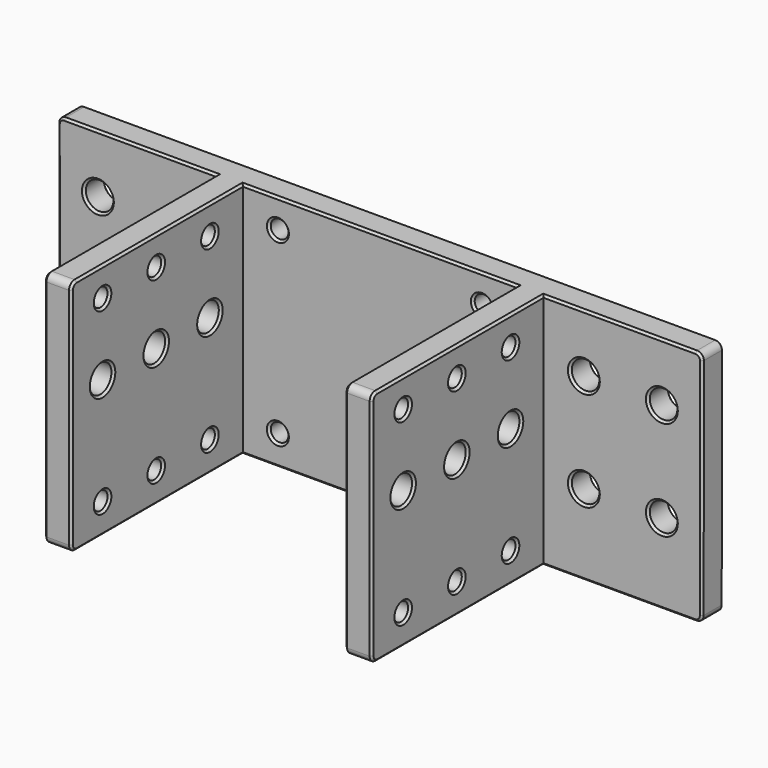
from build123d import *

# Parameters (mm, degrees)
F0_W       = 6.35
F0_H       = 56.2863781022
F1_DEPTH   = 57.15
F0_R       = 3.2639
F0_R_2     = 2.0955
F2_DEPTH   = 6.35
F4_SIZE2   = 1.27
F4_SIZE    = 1.5875
F4_2_SIZE2 = 1.27
F4_2_SIZE  = 1.5875
F4_3_SIZE2 = 1.27
F4_3_SIZE  = 1.5875
F4_4_SIZE2 = 1.27
F4_4_SIZE  = 1.5875
F5_R       = 1.6002
F6_SIZE    = 0.508
F7_R       = 3.2639
F7_R_2     = 2.0955
F8_DEPTH   = 114.9842375546
F9_SIZE    = 0.508


# Not quite as in the source:
# - a feature names something its author has since deleted; it is built from what else it names


with BuildPart() as f1:
    # F0 (on Front) → F1 (new body)
    with BuildSketch(Plane.XZ):
        with Locations((-35.56, 0)):
            Rectangle(F0_W, F0_H)
    extrude(amount=F1_DEPTH)



with BuildPart() as f1b:
    # F0 (on Front) → F1, piece 2 (new body)
    with BuildSketch(Plane.XZ):
        with Locations((35.56, 0)):
            Rectangle(F0_W, F0_H)
    extrude(amount=F1_DEPTH)


with BuildPart() as f1_1:
    add(f1.part)

    add(f1b.part)  # F2 merges F1b
    # F0 (on Front) → F2 (join)
    with BuildSketch(Plane.XZ):
        Polygon((-76.249649699, 28.1431890511), (-76.2, -28.1431890511), (-38.735, -28.1431890511), (-38.735, 28.1431890511), align=None)
        with Locations((-66.7125248495, -9.0931890511)):
            Circle(F0_R, mode=Mode.SUBTRACT)
        with Locations((-48.26, -9.0424341398)):
            Circle(F0_R, mode=Mode.SUBTRACT)
        with Locations((-66.7125248495, 14.4018109489)):
            Circle(F0_R, mode=Mode.SUBTRACT)
        with Locations((-48.26, 14.4525658602)):
            Circle(F0_R, mode=Mode.SUBTRACT)
        Polygon((-32.385, 28.1431890511), (-32.385, -28.1431890511), (0, -28.1431890511), (32.385, -28.1431890511), (32.385, 28.1431890511), (0, 28.1431890511), align=None)
        with Locations((-24.13, -21.0311890511)):
            Circle(F0_R_2, mode=Mode.SUBTRACT)
        with Locations((24.13, -21.0311890511)):
            Circle(F0_R_2, mode=Mode.SUBTRACT)
        with Locations((-24.13, 21.3106109489)):
            Circle(F0_R_2, mode=Mode.SUBTRACT)
        with Locations((24.13, 21.3106109489)):
            Circle(F0_R_2, mode=Mode.SUBTRACT)
        Polygon((38.735, 28.1431890511), (38.735, -28.1431890511), (76.2, -28.1431890511), (76.249649699, 28.1431890511), align=None)
        with Locations((48.26, -9.0424341398)):
            Circle(F0_R, mode=Mode.SUBTRACT)
        with Locations((66.7125248495, -9.0931890511)):
            Circle(F0_R, mode=Mode.SUBTRACT)
        with Locations((48.26, 14.4525658602)):
            Circle(F0_R, mode=Mode.SUBTRACT)
        with Locations((66.7125248495, 14.4018109489)):
            Circle(F0_R, mode=Mode.SUBTRACT)
    extrude(amount=F2_DEPTH)

    # F3: union 

    # F4
    f4_edges = [f1_1.edges().sort_by_distance(p)[0] for p in [
        (22.0345, 0, 21.310611),
    ]]
    f4_side = f1_1.faces().sort_by_distance((22.0345, -3.175, 21.310611))[0]
    chamfer(f4_edges, length=F4_SIZE, length2=F4_SIZE2, reference=f4_side)

    # F4#2
    f4_2_edges = [f1_1.edges().sort_by_distance(p)[0] for p in [
        (-26.2255, 0, 21.310611),
    ]]
    f4_2_side = f1_1.faces().sort_by_distance((-26.2255, -3.175, 21.310611))[0]
    chamfer(f4_2_edges, length=F4_2_SIZE, length2=F4_2_SIZE2, reference=f4_2_side)

    # F4#3
    f4_3_edges = [f1_1.edges().sort_by_distance(p)[0] for p in [
        (22.0345, 0, -21.031189),
    ]]
    f4_3_side = f1_1.faces().sort_by_distance((22.0345, -3.175, -21.031189))[0]
    chamfer(f4_3_edges, length=F4_3_SIZE, length2=F4_3_SIZE2, reference=f4_3_side)

    # F4#4
    f4_4_edges = [f1_1.edges().sort_by_distance(p)[0] for p in [
        (-26.2255, 0, -21.031189),
    ]]
    f4_4_side = f1_1.faces().sort_by_distance((-26.2255, -3.175, -21.031189))[0]
    chamfer(f4_4_edges, length=F4_4_SIZE, length2=F4_4_SIZE2, reference=f4_4_side)

    # F5
    f5_edges = [f1_1.edges().sort_by_distance(p)[0] for p in [
        (76.24965, -3.175, 28.143189),
        (-76.24965, -3.175, 28.143189),
        (76.2, -3.175, -28.143189),
        (-76.2, -3.175, -28.143189),
        (-35.56, -57.15, 28.143189),
        (-35.56, -57.15, -28.143189),
        (35.56, -57.15, 28.143189),
        (35.56, -57.15, -28.143189),
    ]]
    fillet(f5_edges, radius=F5_R)

    # F6
    f6_edges = [f1_1.edges().sort_by_distance(p)[0] for p in [
        (63.448625, 0, 14.401811),
        (44.9961, 0, 14.452566),
        (63.448625, 0, -9.093189),
        (44.9961, 0, -9.042434),
        (-51.5239, 0, 14.452566),
        (-69.976425, 0, 14.401811),
        (-69.976425, 0, -9.093189),
        (-51.5239, 0, -9.042434),
        (76.224824, 0, -0.001412),
        (-56.691519, -6.35, 28.143189),
        (0, -6.35, 28.143189),
        (76.224824, -6.35, -0.001412),
        (0, -6.35, -28.143189),
        (32.385, -30.9499, -28.143189),
        (35.56, -55.5498, -28.143189),
        (38.735, -30.9499, -28.143189),
        (-32.385, -30.9499, -28.143189),
        (56.668105, -6.35, -28.143189),
        (-35.56, -55.5498, -28.143189),
        (74.601211, -3.175, -28.143189),
        (-38.735, -30.9499, -28.143189),
        (0, 0, -28.143189),
        (-56.668105, -6.35, -28.143189),
        (-74.601211, -3.175, -28.143189),
        (56.691519, -6.35, 28.143189),
        (-69.976425, -6.35, 14.401811),
        (-51.5239, -6.35, 14.452566),
        (-69.976425, -6.35, -9.093189),
        (-51.5239, -6.35, -9.042434),
        (-26.2255, -6.35, 21.310611),
        (22.0345, -6.35, 21.310611),
        (-26.2255, -6.35, -21.031189),
        (22.0345, -6.35, -21.031189),
        (44.9961, -6.35, 14.452566),
        (63.448625, -6.35, 14.401811),
        (44.9961, -6.35, -9.042434),
        (63.448625, -6.35, -9.093189),
    ]]
    chamfer(f6_edges, length=F6_SIZE)

    # F7 (on face) → F8 (cut, through all)
    with BuildSketch(Plane.YZ.offset(38.735)):
        with Locations((-47.879, 4.3688109489)):
            Circle(F7_R)
        with Locations((-16.129, 4.3688109489)):
            Circle(F7_R)
        with Locations((-47.879, 21.3106109489)):
            Circle(F7_R_2)
        with Locations((-16.129, 21.3106109489)):
            Circle(F7_R_2)
        with Locations((-32.004, 21.3106109489)):
            Circle(F7_R_2)
        with Locations((-47.879, -21.0311890511)):
            Circle(F7_R_2)
        with Locations((-32.004, -21.0311890511)):
            Circle(F7_R_2)
        with Locations((-16.129, -21.0311890511)):
            Circle(F7_R_2)
        with Locations((-32.004, 4.3688109489)):
            Circle(F7_R)
    extrude(amount=-F8_DEPTH, mode=Mode.SUBTRACT)

    # F9
    f9_edges = [f1_1.edges().sort_by_distance(p)[0] for p in [
        (38.735, -51.1429, 4.368811),
        (38.735, -19.3929, 4.368811),
        (32.385, -51.1429, 4.368811),
        (32.385, -19.3929, 4.368811),
        (-32.385, -51.1429, 4.368811),
        (-32.385, -19.3929, 4.368811),
        (-38.735, -51.1429, 4.368811),
        (-38.735, -19.3929, 4.368811),
        (38.735, -49.9745, 21.310611),
        (38.735, -34.0995, 21.310611),
        (38.735, -18.2245, 21.310611),
        (38.735, -49.9745, -21.031189),
        (38.735, -34.0995, -21.031189),
        (38.735, -18.2245, -21.031189),
        (38.735, -35.2679, 4.368811),
        (32.385, -49.9745, 21.310611),
        (32.385, -49.9745, -21.031189),
        (32.385, -34.0995, 21.310611),
        (32.385, -35.2679, 4.368811),
        (32.385, -18.2245, 21.310611),
        (32.385, -34.0995, -21.031189),
        (32.385, -18.2245, -21.031189),
        (-32.385, -49.9745, -21.031189),
        (-32.385, -49.9745, 21.310611),
        (-32.385, -34.0995, -21.031189),
        (-32.385, -18.2245, -21.031189),
        (-32.385, -35.2679, 4.368811),
        (-32.385, -34.0995, 21.310611),
        (-32.385, -18.2245, 21.310611),
        (-38.735, -49.9745, 21.310611),
        (-38.735, -49.9745, -21.031189),
        (-38.735, -34.0995, 21.310611),
        (-38.735, -35.2679, 4.368811),
        (-38.735, -18.2245, 21.310611),
        (-38.735, -34.0995, -21.031189),
        (-38.735, -18.2245, -21.031189),
    ]]
    chamfer(f9_edges, length=F9_SIZE)


solid = f1_1.part
